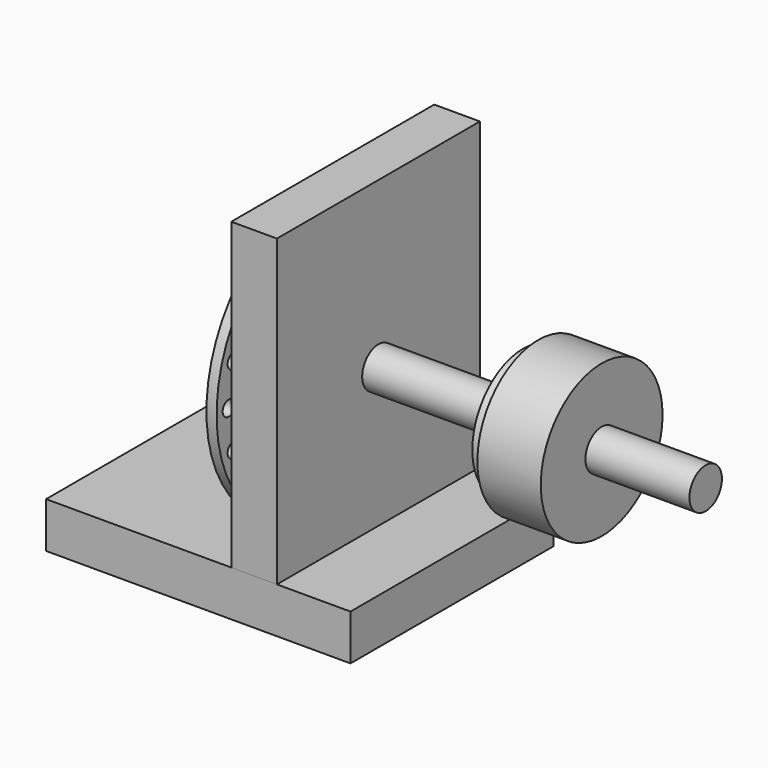
from build123d import *

# Parameters (mm, degrees)
F0_R            = 56
F0_R_2          = 6
F1_DEPTH        = 2
F1_DEPTH_BACK   = 2
F2_R            = 3
F3_DEPTH        = 4.001
F3_COPIES_COUNT = 20
F4_W            = 120
F4_H            = 18
F5_DEPTH        = 50
F5_DEPTH_BACK   = 50
F6_W            = 18
F6_H            = 100
F7_DEPTH        = 120
F8_R            = 5
F9_DEPTH        = 91.001
F10_R           = 8
F11_DEPTH       = 150
F11_DEPTH_BACK  = 12
F13_D           = 4.5
F14_W           = 45
F14_H           = 20
F15_DEPTH       = 3
F17_D           = 4.5
F17_CSINK_D     = 8.96
F17_CSINK_ANGLE = 90
F18_D           = 16
F21_R           = 30
F21_R_2         = 8
F22_DEPTH       = 25
F24_DEPTH       = 10


# Not quite as in the source:
# - a pattern or mirror of a feature is missing from the dataset's text; its kind, count and spacing are read off the source's solid


with BuildPart() as f1:
    # F0 (on Right) → F1 (new body, two sides)
    with BuildSketch(Plane.YZ) as f1_sk:
        Circle(F0_R)
        Circle(F0_R_2, mode=Mode.SUBTRACT)
    extrude(amount=F1_DEPTH)
    extrude(f1_sk.sketch, amount=-F1_DEPTH_BACK)

    # F2 (on face) → F3 (cut, through all)
    with BuildSketch(Plane.YZ.offset(2)):
        with Locations((0, 50)):
            Circle(F2_R)
    f3 = extrude(amount=-F3_DEPTH, mode=Mode.SUBTRACT)

    # F3_copies: F3 ×20 about axis
    f3_copies_axis = Axis((0, 0, 0), (1, 0, 0))
    for i in range(1, F3_COPIES_COUNT):
        add(f3.rotate(f3_copies_axis, i * 360 / F3_COPIES_COUNT), mode=Mode.SUBTRACT)

    # F13 (through all)
    with Locations(Plane(origin=(-2, 0, 0), x_dir=(0, -1, 0), z_dir=(-1, 0, 0))):
        with Locations((-15, 0), (15, 0)):
            Hole(F13_D / 2)


with BuildPart() as f5:
    # F4 (on Front) → F5 (new body, two sides)
    with BuildSketch(Plane.XZ) as f5_sk:
        with Locations((-10, -64)):
            Rectangle(F4_W, F4_H)
    extrude(amount=F5_DEPTH)
    extrude(f5_sk.sketch, amount=-F5_DEPTH_BACK)


with BuildPart() as f7:
    # F6 (on face) → F7 (new body)
    with BuildSketch(Plane.XY.offset(-55)):
        with Locations((12, 0)):
            Rectangle(F6_W, F6_H)
    extrude(amount=F7_DEPTH)

    # F8 (on face) → F9 (cut, through all)
    with BuildSketch(Plane.YZ.offset(21)):
        Circle(F8_R)
    extrude(amount=-F9_DEPTH, mode=Mode.SUBTRACT)


with BuildPart() as f11:
    # F10 (on Right) → F11 (new body, two sides)
    with BuildSketch(Plane.YZ) as f11_sk:
        Circle(F10_R)
    extrude(amount=F11_DEPTH)
    extrude(f11_sk.sketch, amount=-F11_DEPTH_BACK)

    # F23 (on face) → F24 (cut)
    with BuildSketch(Plane(origin=(-12, 0, 0), x_dir=(0, -1, 0), z_dir=(-1, 0, 0))):
        with BuildLine():
            Line((-5.2915026221, 6), (5.2915026221, 6))
            ThreePointArc((5.2915026221, 6), (0, 8), (-5.2915026221, 6))
        make_face()
        with BuildLine():
            ThreePointArc((8, 0), (7.4833147735, 2.8284271247), (6, 5.2915026221))
            Line((6, 5.2915026221), (6, -5.2915026221))
            ThreePointArc((6, -5.2915026221), (7.4833147735, -2.8284271247), (8, 0))
        make_face()
        with BuildLine():
            Line((-6, -5.2915026221), (-6, 5.2915026221))
            ThreePointArc((-6, 5.2915026221), (-8, 0), (-6, -5.2915026221))
        make_face()
        with BuildLine():
            ThreePointArc((-5.2915026221, -6), (0, -8), (5.2915026221, -6))
            Line((5.2915026221, -6), (-5.2915026221, -6))
        make_face()
        with BuildLine():
            ThreePointArc((-5.2915026221, -6), (-5.6568542495, -5.6568542495), (-6, -5.2915026221))
            Line((-6, -5.2915026221), (-6, -6))
            Line((-6, -6), (-5.2915026221, -6))
        make_face()
    extrude(amount=-F24_DEPTH, mode=Mode.SUBTRACT)


with BuildPart() as f15:
    # F14 (on face) → F15 (new body)
    with BuildSketch(Plane(origin=(-2, 0, 0), x_dir=(0, -1, 0), z_dir=(-1, 0, 0))):
        Rectangle(F14_W, F14_H)
    extrude(amount=F15_DEPTH)

    # F17 (through all)
    with Locations(Plane(origin=(-5, 0, 0), x_dir=(0, -1, 0), z_dir=(-1, 0, 0))):
        with Locations((-15, 0), (15, 0)):
            CounterSinkHole(F17_D / 2, F17_CSINK_D / 2, counter_sink_angle=F17_CSINK_ANGLE)

    # F18 (through all)
    with Locations(Plane(origin=(-5, 0, 0), x_dir=(0, -1, 0), z_dir=(-1, 0, 0))):
        with Locations((0, 0)):
            Hole(F18_D / 2)


with BuildPart() as f20:
    # F19 (on Front) → F20 (revolve)
    with BuildSketch(Plane.XZ):
        Polygon((81, 5), (84, 5), (84, 25), (81, 25), (78, 25), (78, 5), align=None)
    revolve(axis=Axis((192.5860950764, 0, 0), (1, 0, 0)))


with BuildPart() as f22:
    # F21 (on face) → F22 (new body)
    with BuildSketch(Plane.YZ.offset(84)):
        Circle(F21_R)
        Circle(F21_R_2, mode=Mode.SUBTRACT)
    extrude(amount=F22_DEPTH)


solid = Compound([f1.part, f5.part, f7.part, f11.part, f15.part, f20.part, f22.part])
